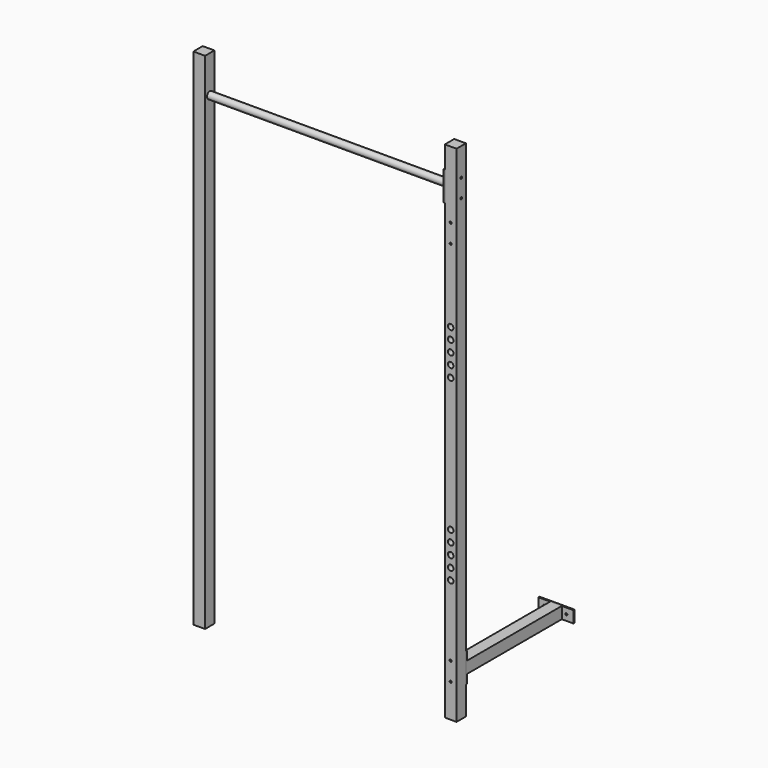
from build123d import *

# Parameters (mm, degrees)
F0_W      = 53.34
F0_H      = 53.34
F1_DEPTH  = 2298.7
F2_W      = 53.34
F2_H      = 40.005
F2_R      = 4.7625
F2_H_2    = 53.34
F3_DEPTH  = 6.35
F4_DEPTH  = 546.1
F5_W      = 160.02
F5_H      = 53.34
F5_R      = 4.7625
F6_DEPTH  = 6.35
F7_DEPTH  = 53.341
F8_W      = 53.34
F8_H      = 133.35
F8_R      = 4.7625
F8_R_2    = 15.875
F9_DEPTH  = 6.35
F10_DEPTH = 1092.2
F11_DEPTH = 106.681
F12_R     = 12.7
F13_DEPTH = 605.791


# Not quite as in the source:
# - a feature names something its author has since deleted; it is built from what else it names


with BuildPart() as f1:
    # F0 (on Top) → F1 (new body)
    with BuildSketch(Plane.XY):
        with Locations((-494.0759591283, 7.5824735198)):
            Rectangle(F0_W, F0_H)
    extrude(amount=F1_DEPTH)


with BuildPart() as f1b:
    # F0 (on Top) → F1, piece 2 (new body)
    with BuildSketch(Plane.XY):
        with Locations((651.4640408717, 7.5824735198)):
            Rectangle(F0_W, F0_H)
    extrude(amount=F1_DEPTH)

    # F2 (on face) → F7 (cut, through all)
    with BuildSketch(Plane(origin=(0, 34.2524735198, 0), x_dir=(-1, 0, 0), z_dir=(0, 1, 0))):
        with Locations((-651.4640408717, 237.1725)):
            Circle(F2_R)
        with Locations((-651.4640408717, 152.4)):
            Circle(F2_R)
        with Locations((-651.4640408717, 1993.9)):
            Circle(F2_R)
        with Locations((-651.4640408717, 1909.1275)):
            Circle(F2_R)
    extrude(amount=-F7_DEPTH, mode=Mode.SUBTRACT)

    # F8 (on face) → F11 (cut, through all)
    with BuildSketch(Plane(origin=(624.7940408717, 0, 0), x_dir=(0, -1, 0), z_dir=(-1, 0, 0))):
        with Locations((-7.5824735198, 2171.7)):
            Circle(F8_R)
        with Locations((-7.5824735198, 2089.15)):
            Circle(F8_R)
    extrude(amount=-F11_DEPTH, mode=Mode.SUBTRACT)

    # F12 (on face) → F13 (cut, through all)
    with BuildSketch(Plane.XZ.offset(19.0875264802)):
        with Locations((651.4640408717, 558.8)):
            Circle(F12_R)
        with Locations((651.4640408717, 609.6)):
            Circle(F12_R)
        with Locations((651.4640408717, 660.4)):
            Circle(F12_R)
        with Locations((651.4640408717, 711.2)):
            Circle(F12_R)
        with Locations((651.4640408717, 762)):
            Circle(F12_R)
        with Locations((651.4640408717, 1371.6)):
            Circle(F12_R)
        with Locations((651.4640408717, 1422.4)):
            Circle(F12_R)
        with Locations((651.4640408717, 1473.2)):
            Circle(F12_R)
        with Locations((651.4640408717, 1524)):
            Circle(F12_R)
        with Locations((651.4640408717, 1574.8)):
            Circle(F12_R)
    extrude(amount=-F13_DEPTH, mode=Mode.SUBTRACT)


with BuildPart() as f3:
    # F2 (on face) → F3 (new body)
    with BuildSketch(Plane(origin=(0, 34.2524735198, 0), x_dir=(-1, 0, 0), z_dir=(0, 1, 0))):
        with Locations((-651.4640408717, 241.45875)):
            Rectangle(F2_W, F2_H)
        with Locations((-651.4640408717, 237.1725)):
            Circle(F2_R, mode=Mode.SUBTRACT)
        with Locations((-651.4640408717, 194.78625)):
            Rectangle(F2_W, F2_H_2)
        with Locations((-651.4640408717, 148.11375)):
            Rectangle(F2_W, F2_H)
        with Locations((-651.4640408717, 152.4)):
            Circle(F2_R, mode=Mode.SUBTRACT)
    extrude(amount=F3_DEPTH)


with BuildPart() as f4:
    # F2 (on face) → F4 (new body)
    with BuildSketch(Plane(origin=(0, 34.2524735198, 0), x_dir=(-1, 0, 0), z_dir=(0, 1, 0))):
        with Locations((-651.4640408717, 194.78625)):
            Rectangle(F2_W, F2_H_2)
    extrude(amount=F4_DEPTH)


with BuildPart() as f6:
    # F5 (on face) → F6 (new body)
    with BuildSketch(Plane(origin=(0, 580.3524735198, 0), x_dir=(-1, 0, 0), z_dir=(0, 1, 0))):
        with Locations((-651.4640408717, 194.78625)):
            Rectangle(F5_W, F5_H)
        with Locations((-698.8772153854, 194.78625)):
            Circle(F5_R, mode=Mode.SUBTRACT)
        with Locations((-596.2894558907, 194.78625)):
            Circle(F5_R, mode=Mode.SUBTRACT)
    extrude(amount=F6_DEPTH)


with BuildPart() as f9:
    # F8 (on face) → F9 (new body)
    with BuildSketch(Plane(origin=(624.7940408717, 0, 0), x_dir=(0, -1, 0), z_dir=(-1, 0, 0))):
        with Locations((-7.5824735198, 2130.425)):
            Rectangle(F8_W, F8_H)
        with Locations((-7.5824735198, 2089.15)):
            Circle(F8_R, mode=Mode.SUBTRACT)
        with Locations((-7.5824735198, 2130.425)):
            Circle(F8_R_2, mode=Mode.SUBTRACT)
        with Locations((-7.5824735198, 2171.7)):
            Circle(F8_R, mode=Mode.SUBTRACT)
    extrude(amount=F9_DEPTH)


with BuildPart() as f10:
    # F8 (on face) → F10 (new body, through all)
    with BuildSketch(Plane(origin=(624.7940408717, 0, 0), x_dir=(0, -1, 0), z_dir=(-1, 0, 0))):
        with Locations((-7.5824735198, 2130.425)):
            Circle(F8_R_2)
    extrude(amount=F10_DEPTH)


solid = Compound([f1.part, f1b.part, f3.part, f4.part, f6.part, f9.part, f10.part])
